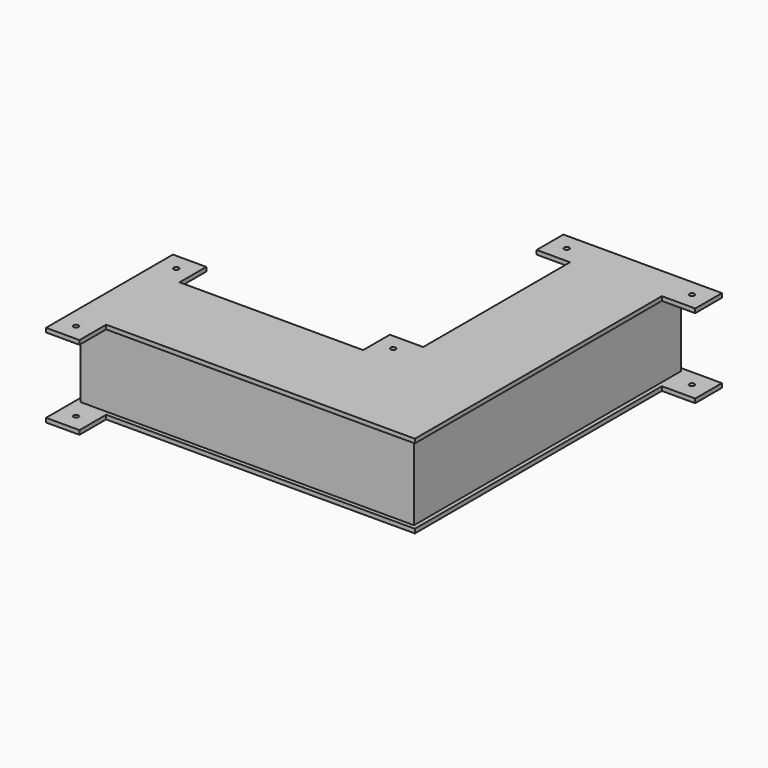
from build123d import *

# Parameters (mm, degrees)
F1_DEPTH = 57.15
F2_R     = 2.8624183912
F2_R_2   = 1.905
F3_DEPTH = 3.175
F4_R     = 1.905
F5_DEPTH = 3.175


with BuildPart() as f1:
    # F0 (on Top) → F1 (new body)
    with BuildSketch(Plane.XY):
        Polygon((-190.5, 0), (-190.5, -63.5), (63.5, -63.5), (63.5, 190.5), (0, 190.5), (0, 0), align=None)
    extrude(amount=F1_DEPTH)

    # F2 (on face) → F3 (join)
    with BuildSketch(Plane(origin=(0, 0, 0), x_dir=(1, 0, 0), z_dir=(0, 0, -1))):
        Polygon((-168.275, -3.175), (-28.575, -3.175), (-28.575, -28.575), (-3.175, -28.575), (-3.175, -168.275), (-28.575, -168.275), (-28.575, -193.675), (-3.175, -193.675), (66.675, -193.675), (92.075, -193.675), (92.075, -168.275), (66.675, -168.275), (66.675, 66.675), (-168.275, 66.675), (-168.275, 92.075), (-193.675, 92.075), (-193.675, 66.675), (-193.675, -3.175), (-193.675, -28.575), (-168.275, -28.575), align=None)
        Polygon((-190.5, 0), (-190.5, 63.5), (63.5, 63.5), (63.5, -190.5), (0, -190.5), (0, 0), align=None, mode=Mode.SUBTRACT)
        with Locations((-15.875, -180.975)):
            Circle(F2_R, mode=Mode.SUBTRACT)
        with Locations((79.375, -180.975)):
            Circle(F2_R_2, mode=Mode.SUBTRACT)
        with Locations((-180.975, -15.875)):
            Circle(F2_R_2, mode=Mode.SUBTRACT)
        with Locations((-180.975, 79.375)):
            Circle(F2_R_2, mode=Mode.SUBTRACT)
        with Locations((-15.875, -15.875)):
            Circle(F2_R_2, mode=Mode.SUBTRACT)
        Polygon((63.5, 63.5), (-190.5, 63.5), (-190.5, 0), (0, 0), (0, -190.5), (63.5, -190.5), align=None)
    extrude(amount=F3_DEPTH)

    # F4 (on face) → F5 (join)
    with BuildSketch(Plane.XY.offset(57.15)):
        Polygon((-28.575, 168.275), (-3.175, 168.275), (-3.175, 28.575), (-28.575, 28.575), (-28.575, 3.175), (-168.275, 3.175), (-168.275, 28.575), (-193.675, 28.575), (-193.675, 3.175), (-193.675, -66.675), (-193.675, -92.075), (-168.275, -92.075), (-168.275, -66.675), (66.675, -66.675), (66.675, 168.275), (92.075, 168.275), (92.075, 193.675), (66.675, 193.675), (-3.175, 193.675), (-28.575, 193.675), align=None)
        with Locations((-180.975, -79.375)):
            Circle(F4_R, mode=Mode.SUBTRACT)
        with Locations((-180.975, 15.875)):
            Circle(F4_R, mode=Mode.SUBTRACT)
        with Locations((-15.875, 15.875)):
            Circle(F4_R, mode=Mode.SUBTRACT)
        with Locations((-15.875, 180.975)):
            Circle(F4_R, mode=Mode.SUBTRACT)
        with Locations((79.375, 180.975)):
            Circle(F4_R, mode=Mode.SUBTRACT)
    extrude(amount=F5_DEPTH)


solid = f1.part
